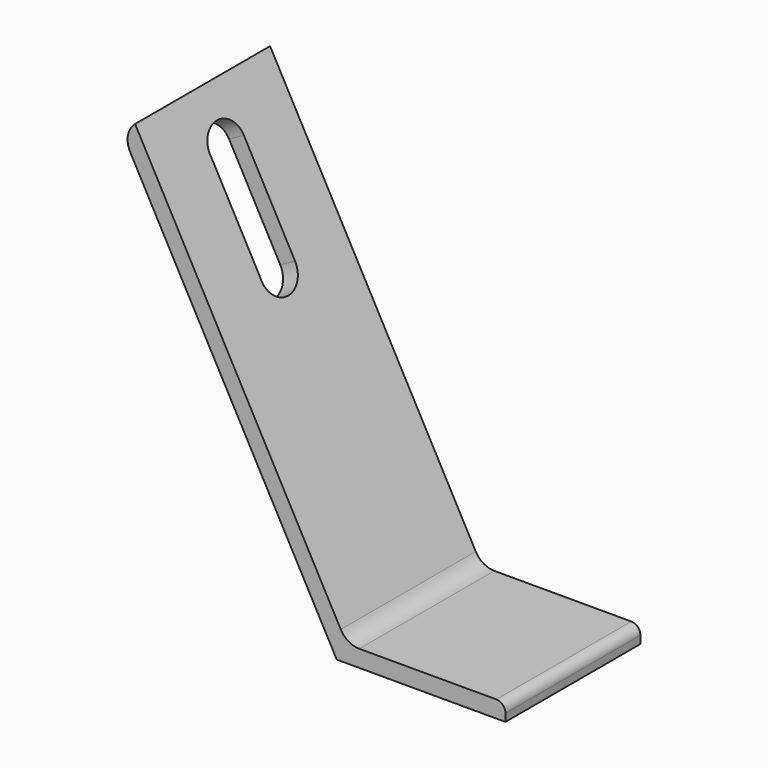
from build123d import *

# Parameters (mm, degrees)
F1_DEPTH    = 40
F2_T1_DEPTH = 40
F2_T3_DEPTH = 64.4948974279
F3_T1_DEPTH = 50.8639610307
F5_DEPTH    = 25


# Not quite as in the source:
# - a fillet or chamfer that OpenCascade refuses, or shapes differently, is made with other operations: its cross-section is extruded or revolved along the edge and cut away or added
# - a feature names something its author has since deleted; it is built from what else it names


with BuildPart() as f1:
    # F0 (on Front) → F1 (new body)
    with BuildSketch(Plane.XZ):
        Polygon((-51.3135007212, 94.3231601012), (-3, 5.5145230071), (0, 0), (40, 0), (40, 4), (2.3775297152, 4), (-47.7997987259, 96.2346773752), align=None)
    extrude(amount=F1_DEPTH)

    # F2: fillet of radius 5 on 2 edges, made by hand

    # F2_s2 → F2_t1 (join)
    with BuildSketch(Plane.XZ):
        with BuildLine():
            ThreePointArc((5.3494418593, 4), (2.7947386439, 4.7019200239), (0.9573143652, 6.6106034076))
            Line((0.9573143652, 6.6106034076), (2.3775297152, 4))
            Line((2.3775297152, 4), (5.3494418593, 4))
        make_face()
    extrude(amount=F2_T1_DEPTH)

    # F2_s4 → F2_t3 (cut)
    with BuildSketch(Plane.XZ.offset(-12.2474487139)):
        with BuildLine():
            ThreePointArc((-47.7997987259, 96.2346773752), (-49.4935666702, 93.3361748844), (-48.9723797433, 90.019771603))
            Line((-48.9723797433, 90.019771603), (-51.3135007212, 94.3231601012))
            Line((-51.3135007212, 94.3231601012), (-47.7997987259, 96.2346773752))
        make_face()
    extrude(amount=F2_T3_DEPTH, mode=Mode.SUBTRACT)

    # F3: fillet of radius 2.1727922061 on 2 edges, made by hand

    # F3_s2 → F3_t1 (cut)
    with BuildSketch(Plane.XZ.offset(-5.4319805153)):
        with BuildLine():
            ThreePointArc((37.8272077939, 4), (39.3636038969, 3.3636038969), (40, 1.8272077939))
            Line((40, 1.8272077939), (40, 4))
            Line((40, 4), (37.8272077939, 4))
        make_face()
    extrude(amount=F3_T1_DEPTH, mode=Mode.SUBTRACT)

    # F4 (on face) → F5 (cut)
    with BuildSketch(Plane(origin=(3.5137019952, 0, 1.9115172739), x_dir=(0, 1, 0), z_dir=(0.8784254988, 0, 0.4778793185))):
        with BuildLine():
            Line((-15, 69.8649734259), (-15, 95.260605216))
            ThreePointArc((-15, 95.260605216), (-19.6685312037, 100.2496059614), (-24.9560513748, 95.9220844447))
            Line((-24.9560513748, 95.9220844447), (-24.9560513748, 94.5991259873))
            Line((-24.9560513748, 94.5991259873), (-24.9560513748, 70.5264526546))
            ThreePointArc((-24.9560513748, 70.5264526546), (-20.3314687963, 64.8759726805), (-15, 69.8649734259))
        make_face()
        with BuildLine():
            Line((-24.9560513748, 94.5991259873), (-24.9560513748, 95.9220844447))
            ThreePointArc((-24.9560513748, 95.9220844447), (-25, 95.260605216), (-24.9560513748, 94.5991259873))
        make_face()
    extrude(amount=-F5_DEPTH, mode=Mode.SUBTRACT)


solid = f1.part
